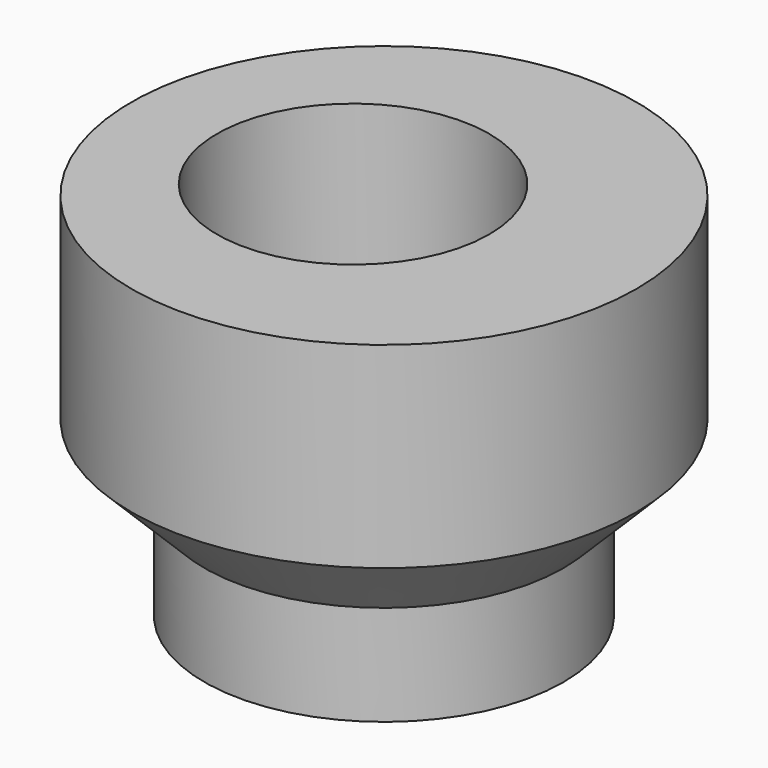
from build123d import *

# Parameters (mm, degrees)
F0_W          = 6.4
F0_H          = 3.175
F2_S5_R       = 6.4
F2_T6_DEPTH   = 14
F3_R          = 4.85
F4_DEPTH      = 25
F4_DEPTH_BACK = 25


# Not quite as in the source:
# - a fillet or chamfer that OpenCascade refuses, or shapes differently, is made with other operations: its cross-section is extruded or revolved along the edge and cut away or added


with BuildPart() as f1:
    # F0 (on Front) → F1 (revolve)
    with BuildSketch(Plane.XZ):
        with Locations((3.2, 0)):
            Rectangle(F0_W, F0_H)
        Polygon((0, 1.5875), (6.4, 1.5875), (9, 1.5875), (9, 11.5875), (0, 11.5875), align=None)
    revolve(axis=Axis((0, 0, 6.5875), (0, 0, -1)))

    # F2: chamfer of 3 on 1 edges, made by hand


with BuildPart() as f2_tool2:
    # F2_s3 → F2_t4 (revolve)
    with BuildSketch(Plane.XZ):
        Polygon((6, 1.5875), (9, 4.5875), (9, 1.5875), align=None)
    revolve(axis=Axis((0, 0, 1.5875), (0, 0, -1)))

    # F2_s5 → F2_t6 (cut, symmetric)
    with BuildSketch(Plane.XY.offset(3.1)):
        Circle(F2_S5_R)
    extrude(amount=F2_T6_DEPTH, both=True, mode=Mode.SUBTRACT)


with BuildPart() as f1_1:
    add(f1.part)

    # F2_t1: cut F2_tool2
    add(f2_tool2.part, mode=Mode.SUBTRACT)

    # F3 (on Top) → F4 (cut, two sides)
    with BuildSketch(Plane.XY) as f4_sk:
        with Locations((-1.1, 0)):
            Circle(F3_R)
    extrude(amount=-F4_DEPTH, mode=Mode.SUBTRACT)
    extrude(f4_sk.sketch, amount=F4_DEPTH_BACK, mode=Mode.SUBTRACT)


solid = f1_1.part
